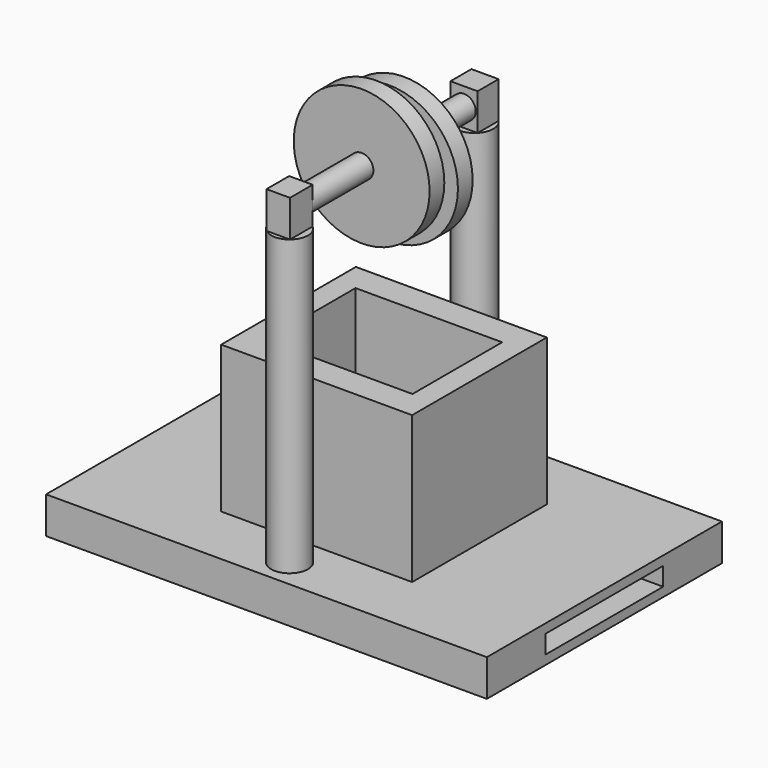
from build123d import *

# Parameters (mm, degrees)
F0_W      = 152.4
F0_H      = 12.7
F1_DEPTH  = 101.6
F3_DEPTH  = 127
F4_W      = 66.0289544821
F4_H      = 58.2000215709
F5_DEPTH  = 50.8
F6_W      = 50.7049728394
F6_H      = 38.7546804905
F7_DEPTH  = 60.452
F8_R      = 6.3611309163
F9_DEPTH  = 101.6
F10_R     = 6.5311843642
F11_DEPTH = 101.6
F12_W     = 8.1331080545
F12_H     = 9.7830720897
F14_DEPTH = 12.7
F13_W     = 9.3966365277
F13_H     = 9.0735163396
F15_DEPTH = 12.7
F16_R     = 4.0494761519
F17_DEPTH = 76.2
F19_R     = 23.756550032
F20_DEPTH = 6.35
F21_R     = 6.35
F22_DEPTH = 3.302
F23_R     = 23.495
F24_DEPTH = 6.35


with BuildPart() as f1:
    # F0 (on Front) → F1 (new body)
    with BuildSketch(Plane.XZ):
        with Locations((76.2, 6.35)):
            Rectangle(F0_W, F0_H)
    extrude(amount=-F1_DEPTH)

    # F2 (on face) → F3 (cut)
    with BuildSketch(Plane.YZ.offset(152.4)):
        Polygon((76.2, 3.175), (76.2, 6.35), (76.2, 9.525), (25.4, 9.525), (25.4, 6.35), (25.4, 3.175), align=None)
    extrude(amount=-F3_DEPTH, mode=Mode.SUBTRACT)

    # F4 (on face) → F5 (join)
    with BuildSketch(Plane.XY.offset(12.7)):
        with Locations((76.2, 50.8)):
            Rectangle(F4_W, F4_H)
    extrude(amount=F5_DEPTH)

    # F6 (on face) → F7 (cut)
    with BuildSketch(Plane.XY.offset(63.5)):
        with Locations((76.2, 50.8)):
            Rectangle(F6_W, F6_H)
    extrude(amount=-F7_DEPTH, mode=Mode.SUBTRACT)


with BuildPart() as f9:
    # F8 (on face) → F9 (new body)
    with BuildSketch(Plane.XY.offset(12.7)):
        with Locations((76.2, 9.9855083972)):
            Circle(F8_R)
    extrude(amount=F9_DEPTH)


with BuildPart() as f11:
    # F10 (on face) → F11 (new body)
    with BuildSketch(Plane.XY.offset(12.7)):
        with Locations((76.2, 89.9265035987)):
            Circle(F10_R)
    extrude(amount=F11_DEPTH)


with BuildPart() as f14:
    # F12 (on face) → F14 (new body)
    with BuildSketch(Plane.XY.offset(114.3)):
        with Locations((76.2, 9.9855083972)):
            Rectangle(F12_W, F12_H)
    extrude(amount=F14_DEPTH)


with BuildPart() as f15:
    # F13 (on face) → F15 (new body)
    with BuildSketch(Plane.XY.offset(114.3)):
        with Locations((76.2, 89.9265035987)):
            Rectangle(F13_W, F13_H)
    extrude(amount=F15_DEPTH)


with BuildPart() as f17:
    # F16 (on face) → F17 (new body)
    with BuildSketch(Plane.XZ.offset(-85.3897454289)):
        with Locations((76.2, 120.65)):
            Circle(F16_R)
    extrude(amount=F17_DEPTH)


with BuildPart() as f20:
    # F19 (on offset) → F20 (new body)
    with BuildSketch(Plane.XZ.offset(-50.8)):
        with Locations((78.0054554343, 118.2057708502)):
            Circle(F19_R)
    extrude(amount=-F20_DEPTH)


with BuildPart() as f22:
    # F21 (on face) → F22 (new body)
    with BuildSketch(Plane.XZ.offset(-50.8)):
        with Locations((76.2, 120.65)):
            Circle(F21_R)
    extrude(amount=F22_DEPTH)


with BuildPart() as f24:
    # F23 (on face) → F24 (new body)
    with BuildSketch(Plane.XZ.offset(-47.498)):
        with Locations((76.2, 120.65)):
            Circle(F23_R)
    extrude(amount=F24_DEPTH)


solid = Compound([f1.part, f9.part, f11.part, f14.part, f15.part, f17.part, f20.part, f22.part, f24.part])
